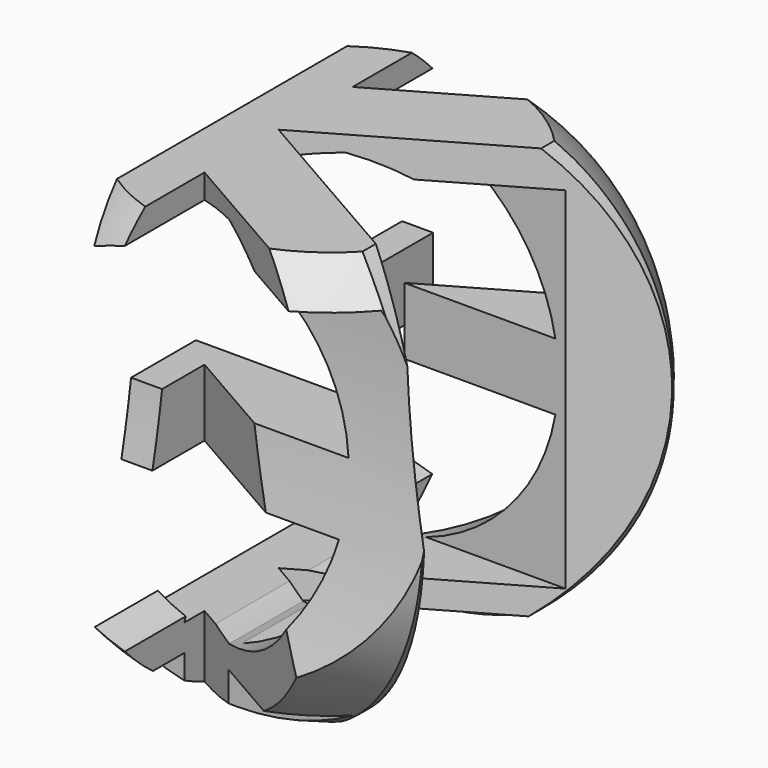
from build123d import *

# Parameters (mm, degrees)
F6_DEPTH  = 48.9
F8_DEPTH  = 73.9
F10_DEPTH = 48.9


# Not quite as in the source:
# - a feature names something its author has since deleted; it is built from what else it names


with BuildPart() as f1:
    # F0 (on Front) → F1 (revolve)
    with BuildSketch(Plane.XZ):
        with BuildLine():
            Line((0, 22.6339450173), (20, 22.6339450173))
            ThreePointArc((20, 22.6339450173), (0, 42.6339450173), (-20, 22.6339450173))
            Line((-20, 22.6339450173), (0, 22.6339450173))
        make_face()
    revolve(axis=Axis((-10, 0, 22.6339450173), (1, 0, 0)))

    # F5 (on offset) → F6 (cut)
    with BuildSketch(Plane.XY.offset(43.3)):
        with BuildLine():
            Line((-11.943612595, -16.0421357113), (-11.943612595, 16.0421357113))
            ThreePointArc((-11.943612595, 16.0421357113), (-20, 0), (-11.943612595, -16.0421357113))
        make_face()
        with BuildLine():
            Line((-3.943612595, -16.0421357113), (-11.943612595, -16.0421357113))
            ThreePointArc((-11.943612595, -16.0421357113), (0, -20), (11.943612595, -16.0421357113))
            Line((11.943612595, -16.0421357113), (-3.943612595, -6.9189172936))
            Line((-3.943612595, -6.9189172936), (-3.943612595, -16.0421357113))
        make_face()
        with BuildLine():
            ThreePointArc((20, 0), (19.0478295378, 6.0975560595), (16.2819810101, 11.6145208418))
            Line((16.2819810101, 11.6145208418), (-3.943612595, 0))
            Line((-3.943612595, 0), (16.2819810101, -11.6145208418))
            ThreePointArc((16.2819810101, -11.6145208418), (19.0478295378, -6.0975560595), (20, 0))
        make_face()
        with BuildLine():
            ThreePointArc((11.943612595, 16.0421357113), (0, 20), (-11.943612595, 16.0421357113))
            Line((-11.943612595, 16.0421357113), (-3.943612595, 16.0421357113))
            Line((-3.943612595, 16.0421357113), (-3.943612595, 6.9189172936))
            Line((-3.943612595, 6.9189172936), (11.943612595, 16.0421357113))
        make_face()
    extrude(amount=-F6_DEPTH, mode=Mode.SUBTRACT)

    # F7 (on offset) → F8 (cut)
    with BuildSketch(Plane.XZ.offset(22)):
        with BuildLine():
            ThreePointArc((-8.6470612384, 40.6680330713), (-4.4108839223, 42.0352124388), (0, 42.6339450173))
            ThreePointArc((0, 42.6339450173), (-4.4338605594, 42.1362751484), (-8.6470612384, 40.6680330713))
        make_face()
        with BuildLine():
            ThreePointArc((-8.6470612384, 4.5998569633), (-4.4338605594, 3.1316148863), (0, 2.6339450173))
            ThreePointArc((0, 2.6339450173), (-4.4147481905, 3.2156806169), (-8.6470612384, 4.5998569633))
        make_face()
        with BuildLine():
            ThreePointArc((0, 2.6339450173), (14.1421356237, 8.4918093936), (20, 22.6339450173))
            ThreePointArc((20, 22.6339450173), (14.1421356237, 36.7760806411), (0, 42.6339450173))
            ThreePointArc((0, 42.6339450173), (16.2134145309, 22.6339450173), (0, 2.6339450173))
        make_face()
        with BuildLine():
            Line((-6.3060164348, 35.1435851435), (-8.6470612384, 40.6680330713))
            ThreePointArc((-8.6470612384, 40.6680330713), (-20, 22.6339450173), (-8.6470612384, 4.5998569633))
            Line((-8.6470612384, 4.5998569633), (-6.2630078533, 10.105879966))
            ThreePointArc((-6.2630078533, 10.105879966), (-3.4533212877, 9.1542824914), (-0.5259139232, 8.6745299795))
            ThreePointArc((-0.5259139232, 8.6745299795), (6.4095593768, 12.8665228434), (9.9953882922, 20.1339450173))
            Line((9.9953882922, 20.1339450173), (-6.2630078533, 20.1339450173))
            Line((-6.2630078533, 20.1339450173), (-6.2630078533, 25.1339450173))
            Line((-6.2630078533, 25.1339450173), (9.9953882922, 25.1339450173))
            ThreePointArc((9.9953882922, 25.1339450173), (6.4166339458, 32.3936562253), (-0.5056881537, 36.587979323))
            ThreePointArc((-0.5056881537, 36.587979323), (-3.4625761579, 36.093571181), (-6.3060164348, 35.1435851435))
        make_face()
    extrude(amount=-F8_DEPTH, mode=Mode.SUBTRACT)

    # F9 (on offset) → F10 (cut)
    with BuildSketch(Plane.YZ.offset(22)):
        with BuildLine():
            ThreePointArc((-14.5121786365, 36.3960913333), (-13.8048288932, 37.1055274888), (-13.0628413392, 37.7786528767))
            Line((-13.0628413392, 37.7786528767), (-14.5121786365, 37.7786528767))
            Line((-14.5121786365, 37.7786528767), (-14.5121786365, 36.3960913333))
        make_face()
        with BuildLine():
            Line((-6.8110743198, 3.0763908625), (-6.8110743198, 3.8294437846))
            ThreePointArc((-6.8110743198, 3.8294437846), (-7.8226272385, 4.2272477827), (-8.8110743198, 4.6794199796))
            Line((-8.8110743198, 4.6794199796), (-8.8110743198, 3.0763908625))
            Line((-8.8110743198, 3.0763908625), (-6.8110743198, 3.0763908625))
        make_face()
        with BuildLine():
            Line((10.5821458962, 1.4693343882), (10.5821458962, 5.6628464014))
            ThreePointArc((10.5821458962, 5.6628464014), (9.5977452348, 5.0873417447), (8.5821458962, 4.5688745271))
            Line((8.5821458962, 4.5688745271), (8.5821458962, 1.4693343882))
            Line((8.5821458962, 1.4693343882), (10.5821458962, 1.4693343882))
        make_face()
        with BuildLine():
            Line((-14.5121786365, 35.1386720749), (-14.5121786365, 36.3960913333))
            ThreePointArc((-14.5121786365, 36.3960913333), (-19.9964093785, 23.0129067158), (-15.0231970267, 9.4315379983))
            ThreePointArc((-15.0231970267, 9.4315379983), (-11.3953060336, 22.0590998115), (-10.1536539841, 35.1386720749))
            Line((-10.1536539841, 35.1386720749), (-14.5121786365, 35.1386720749))
        make_face()
        with BuildLine():
            Line((-4.193781408, 37.7786528767), (13.0628413392, 37.7786528767))
            ThreePointArc((13.0628413392, 37.7786528767), (0, 42.6339450173), (-13.0628413392, 37.7786528767))
            Line((-13.0628413392, 37.7786528767), (-4.193781408, 37.7786528767))
        make_face()
        with BuildLine():
            ThreePointArc((14.4385592904, 8.7945806672), (18.5576289677, 15.176438256), (20, 22.6339450173))
            ThreePointArc((20, 22.6339450173), (18.5774537105, 30.041928119), (14.5121786365, 36.3960913333))
            Line((14.5121786365, 36.3960913333), (14.5121786365, 35.1386720749))
            Line((14.5121786365, 35.1386720749), (14.4385592904, 35.1386720749))
            Line((14.4385592904, 35.1386720749), (14.4385592904, 8.9291743934))
            Line((14.4385592904, 8.9291743934), (14.4385592904, 8.7945806672))
        make_face()
        with BuildLine():
            Line((-8.8005206947, 8.9291743934), (8.4385592904, 8.9291743934))
            Line((8.4385592904, 8.9291743934), (8.4385592904, 35.1386720749))
            Line((8.4385592904, 35.1386720749), (-4.1536419204, 35.1386720749))
            ThreePointArc((-4.1536419204, 35.1386720749), (-5.337064627, 21.8318011111), (-8.8005206947, 8.9291743934))
        make_face()
        with BuildLine():
            ThreePointArc((-6.8110743198, 3.8294437846), (0.9596161149, 2.6569798596), (8.5821458962, 4.5688745271))
            Line((8.5821458962, 4.5688745271), (8.5821458962, 6.9291743934))
            Line((8.5821458962, 6.9291743934), (-6.8110743198, 6.9291743934))
            Line((-6.8110743198, 6.9291743934), (-6.8110743198, 3.8294437846))
        make_face()
        with BuildLine():
            Line((-8.8110743198, 6.9291743934), (-9.5599580869, 6.9291743934))
            Line((-9.5599580869, 6.9291743934), (-12.3838677177, 6.9291743934))
            ThreePointArc((-12.3838677177, 6.9291743934), (-10.6570043035, 5.7097534775), (-8.8110743198, 4.6794199796))
            Line((-8.8110743198, 4.6794199796), (-8.8110743198, 6.9291743934))
        make_face()
    extrude(amount=-F10_DEPTH, mode=Mode.SUBTRACT)


solid = f1.part
